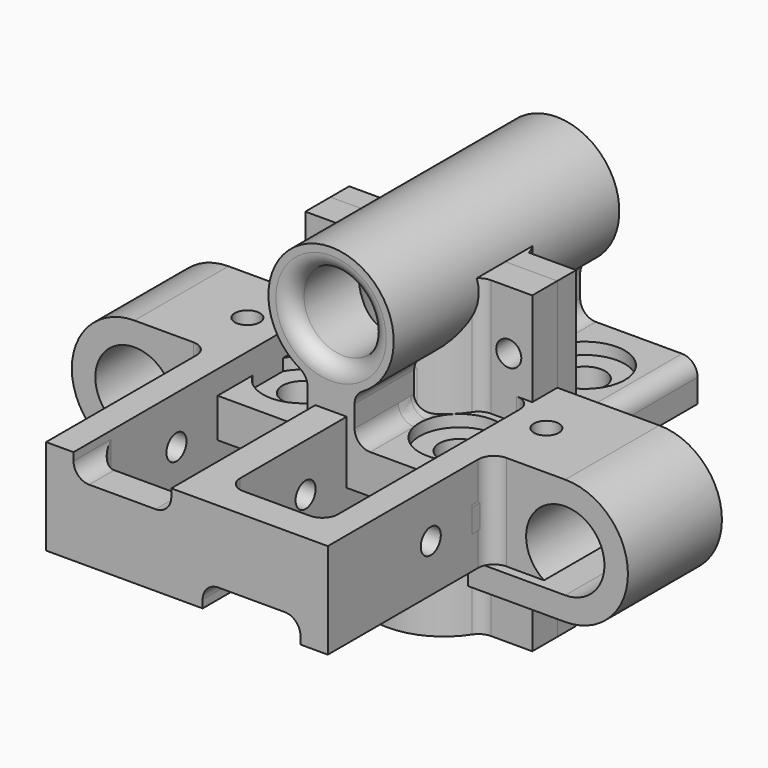
from build123d import *

# Parameters (mm, degrees)
F0_W           = 36
F0_H           = 36
F0_R           = 2.6
F1_DEPTH       = 5
F2_R           = 5.1
F3_DEPTH       = 1.5
F4_R           = 5.05
F5_DEPTH       = 18
F5_DEPTH_BACK  = 18
F6_R           = 2
F8_DEPTH       = 20
F8_DEPTH_BACK  = 20
F11_DEPTH      = 1
F13_DEPTH      = 20
F13_DEPTH_BACK = 20
F9_R           = 1.6
F14_DEPTH      = 10
F16_DEPTH      = 15
F17_W          = 3.5
F17_H          = 12.2
F18_DEPTH      = 22
F20_DEPTH      = 4
F21_DEPTH      = 30
F22_R          = 1.6
F23_DEPTH      = 25
F23_DEPTH_BACK = 25
F24_R          = 2
F25_R          = 1.6
F26_DEPTH      = 17.1


with BuildPart() as f1:
    # F0 (on Top) → F1 (new body)
    with BuildSketch(Plane.XY):
        Rectangle(F0_W, F0_H)
        with Locations((-10, -10)):
            Circle(F0_R, mode=Mode.SUBTRACT)
        with Locations((10, -10)):
            Circle(F0_R, mode=Mode.SUBTRACT)
        with Locations((-10, 10)):
            Circle(F0_R, mode=Mode.SUBTRACT)
        with Locations((10, 10)):
            Circle(F0_R, mode=Mode.SUBTRACT)
    extrude(amount=F1_DEPTH)

    # F2 (on face) → F3 (cut)
    with BuildSketch(Plane.XY.offset(5)):
        with Locations((-10, 10)):
            Circle(F2_R)
        with Locations((-10, -10)):
            Circle(F2_R)
        with Locations((10, 10)):
            Circle(F2_R)
        with Locations((10, -10)):
            Circle(F2_R)
    extrude(amount=-F3_DEPTH, mode=Mode.SUBTRACT)

    # F4 (on Front) → F5 (join, two sides)
    with BuildSketch(Plane.XZ) as f5_sk:
        with BuildLine():
            Line((-3, 11), (-3, 5))
            Line((-3, 5), (3, 5))
            Line((3, 5), (3, 11))
            ThreePointArc((3, 11), (0, 26.4161984871), (-3, 11))
        make_face()
        with Locations((0, 18.4161984871)):
            Circle(F4_R, mode=Mode.SUBTRACT)
    extrude(amount=F5_DEPTH)
    extrude(f5_sk.sketch, amount=-F5_DEPTH_BACK)

    # F6
    f6_edges = [f1.edges().sort_by_distance(p)[0] for p in [
        (-5.05, -18, 18.416198),
        (-3, 0, 5),
        (3, 0, 5),
        (3, 0, 11),
        (-3, 0, 11),
        (-5.05, 18, 18.416198),
        (-18, 0, 5),
        (18, 0, 5),
    ]]
    fillet(f6_edges, radius=F6_R)


with BuildPart() as f8:
    # F7 (on Top) → F8 (new body, two sides)
    with BuildSketch(Plane.XY) as f8_sk:
        with BuildLine():
            ThreePointArc((-6.05, 0), (0, 6.05), (6.05, 0))
            Line((6.05, 0), (9, 0))
            Line((9, 0), (14.4852813742, 0))
            Line((14.4852813742, 0), (14.4852813742, 3))
            Line((14.4852813742, 3), (8.4852813742, 3))
            ThreePointArc((8.4852813742, 3), (0, 9), (-8.4852813742, 3))
            Line((-8.4852813742, 3), (-14.4852813742, 3))
            Line((-14.4852813742, 3), (-14.4852813742, 0))
            Line((-14.4852813742, 0), (-9, 0))
            Line((-9, 0), (-6.05, 0))
        make_face()
    extrude(amount=F8_DEPTH)
    extrude(f8_sk.sketch, amount=-F8_DEPTH_BACK)

    # F10 (on face) → F11 (cut)
    with BuildSketch(Plane(origin=(0, 3, 0), x_dir=(-1, 0, 0), z_dir=(0, 1, 0))):
        Polygon((11.4852813742, -9.2668384925), (8.6852813742, -10.8834192463), (8.6852813742, -14.1165807537), (11.4852813742, -15.7331615075), (14.2852813742, -14.1165807537), (14.2852813742, -10.8834192463), align=None)
        Polygon((8.6852813742, 14.1165807537), (8.6852813742, 10.8834192463), (11.4852813742, 9.2668384925), (14.2852813742, 10.8834192463), (14.2852813742, 14.1165807537), (11.4852813742, 15.7331615075), align=None)
        Polygon((-14.2852813742, 10.8834192463), (-11.4852813742, 9.2668384925), (-8.6852813742, 10.8834192463), (-8.6852813742, 14.1165807537), (-11.4852813742, 15.7331615075), (-14.2852813742, 14.1165807537), align=None)
        Polygon((-11.4852813742, -15.7331615075), (-8.6852813742, -14.1165807537), (-8.6852813742, -10.8834192463), (-11.4852813742, -9.2668384925), (-14.2852813742, -10.8834192463), (-14.2852813742, -14.1165807537), align=None)
    extrude(amount=-F11_DEPTH, mode=Mode.SUBTRACT)


with BuildPart() as f13:
    # F12 (on Top) → F13 (new body, two sides)
    with BuildSketch(Plane.XY) as f13_sk:
        with BuildLine():
            ThreePointArc((6.05, 0), (0, -6.05), (-6.05, 0))
            Line((-6.05, 0), (-14.4852813742, 0))
            Line((-14.4852813742, 0), (-14.4852813742, -4))
            Line((-14.4852813742, -4), (-8.0622577483, -4))
            ThreePointArc((-8.0622577483, -4), (0, -9), (8.0622577483, -4))
            Line((8.0622577483, -4), (14.4852813742, -4))
            Line((14.4852813742, -4), (14.4852813742, 0))
            Line((14.4852813742, 0), (6.05, 0))
        make_face()
    extrude(amount=F13_DEPTH)
    extrude(f13_sk.sketch, amount=-F13_DEPTH_BACK)


with BuildPart() as f14_tool:
    # F9 (on face) → F14 (new body)
    with BuildSketch(Plane(origin=(0, 3, 0), x_dir=(-1, 0, 0), z_dir=(0, 1, 0))):
        with Locations((11.4852813742, -12.5)):
            Circle(F9_R)
        with Locations((11.4852813742, 12.5)):
            Circle(F9_R)
        with Locations((-11.4852813742, -12.5)):
            Circle(F9_R)
        with Locations((-11.4852813742, 12.5)):
            Circle(F9_R)
    extrude(amount=-F14_DEPTH)


with BuildPart() as f8_1:
    add(f8.part)

    # F14: cut by f14_tool
    add(f14_tool.part, mode=Mode.SUBTRACT)


with BuildPart() as f13_1:
    add(f13.part)

    # F14: cut by f14_tool
    add(f14_tool.part, mode=Mode.SUBTRACT)

    # F15 (on Front) → F16 (join)
    with BuildSketch(Plane.XZ):
        with BuildLine():
            ThreePointArc((24.7870680067, -4.2), (28.9142135624, 4.7958315233), (27.5, -5))
            Line((27.5, -5), (15.0852813742, -5))
            Line((15.0852813742, -5), (15.0852813742, -8))
            Line((15.0852813742, -8), (27.5, -8))
            ThreePointArc((27.5, -8), (35.5, 0), (27.5, 8))
            ThreePointArc((27.5, 8), (20.5143003214, 3.8987177379), (20.6911821878, -4.2))
            Line((20.6911821878, -4.2), (24.7870680067, -4.2))
        make_face()
        with BuildLine():
            Line((14.4852813742, -4.2), (20.6911821878, -4.2))
            ThreePointArc((20.6911821878, -4.2), (20.5143003214, 3.8987177379), (27.5, 8))
            Line((27.5, 8), (14.4852813742, 8))
            Line((14.4852813742, 8), (14.4852813742, -4.2))
        make_face()
        with BuildLine():
            Line((-14.4852813742, -4.2), (-14.4852813742, 8))
            Line((-14.4852813742, 8), (-27.5, 8))
            ThreePointArc((-27.5, 8), (-20.5143003214, 3.8987177379), (-20.6911821878, -4.2))
            Line((-20.6911821878, -4.2), (-14.4852813742, -4.2))
        make_face()
        with BuildLine():
            ThreePointArc((-20.6911821878, -4.2), (-20.5143003214, 3.8987177379), (-27.5, 8))
            ThreePointArc((-27.5, 8), (-35.5, 0), (-27.5, -8))
            Line((-27.5, -8), (-15.0852813742, -8))
            Line((-15.0852813742, -8), (-15.0852813742, -5))
            Line((-15.0852813742, -5), (-27.5, -5))
            ThreePointArc((-27.5, -5), (-28.9142135624, 4.7958315233), (-24.7870680067, -4.2))
            Line((-24.7870680067, -4.2), (-20.6911821878, -4.2))
        make_face()
    extrude(amount=F16_DEPTH)

    # F17 (on face) → F18 (join)
    with BuildSketch(Plane.XZ.offset(15)):
        with Locations((16.2352813742, 1.9)):
            Rectangle(F17_W, F17_H)
        with Locations((-16.2352813742, 1.9)):
            Rectangle(F17_W, F17_H)
    extrude(amount=F18_DEPTH)

    # F19 (on face) → F20 (join)
    with BuildSketch(Plane.XZ.offset(37)):
        Polygon((17.9852813742, -4.2), (17.9852813742, 8), (2, 8), (2, -1.2), (14.4852813742, -1.2), (14.4852813742, -4.2), align=None)
        Polygon((2, -1.2), (2, 8), (-2, 8), (-2, 5), (-2, -4.2), (2, -4.2), align=None)
        Polygon((-2, -4.2), (-2, 5), (-14.4852813742, 5), (-14.4852813742, 8), (-17.9852813742, 8), (-17.9852813742, -4.2), align=None)
    extrude(amount=F20_DEPTH)

    # F19 (on face) → F21 (join)
    with BuildSketch(Plane.XZ.offset(37)):
        Polygon((2, -1.2), (2, 8), (-2, 8), (-2, 5), (-2, -4.2), (2, -4.2), align=None)
    extrude(amount=-F21_DEPTH)

    # F22 (on Right) → F23 (cut, two sides)
    with BuildSketch(Plane.YZ) as f23_sk:
        with Locations((-24.5680958033, 1.9)):
            Circle(F22_R)
    extrude(amount=F23_DEPTH, mode=Mode.SUBTRACT)
    extrude(f23_sk.sketch, amount=-F23_DEPTH_BACK, mode=Mode.SUBTRACT)

    # F24
    f24_edges = [f13_1.edges().sort_by_distance(p)[0] for p in [
        (0, -9, 8),
        (-2, -8.774964, 1.9),
        (2, -8.774964, 1.9),
        (0, -9, -4.2),
        (14.485281, -4, 1.9),
        (8.062258, -4, 0),
        (-8.062258, -4, 0),
        (-14.485281, -4, 1.9),
        (2, -37, 3.4),
        (14.485281, -37, 3.4),
        (-2, -37, 0.4),
        (-14.485281, -37, 0.4),
        (-2, -39, 5),
        (2, -39, -1.2),
        (14.485281, -39, -1.2),
        (-14.485281, -39, 5),
        (17.985281, -15, 1.9),
        (-17.985281, -15, 1.9),
    ]]
    fillet(f24_edges, radius=F24_R)

    # F25 (on face) → F26 (cut)
    with BuildSketch(Plane(origin=(0, 0, -8), x_dir=(1, 0, 0), z_dir=(0, 0, -1))):
        with Locations((-19.0852813742, 7.5)):
            Circle(F25_R)
        with Locations((19.0852813742, 7.5)):
            Circle(F25_R)
    extrude(amount=-F26_DEPTH, mode=Mode.SUBTRACT)


solid = Compound([f1.part, f8_1.part, f13_1.part])
